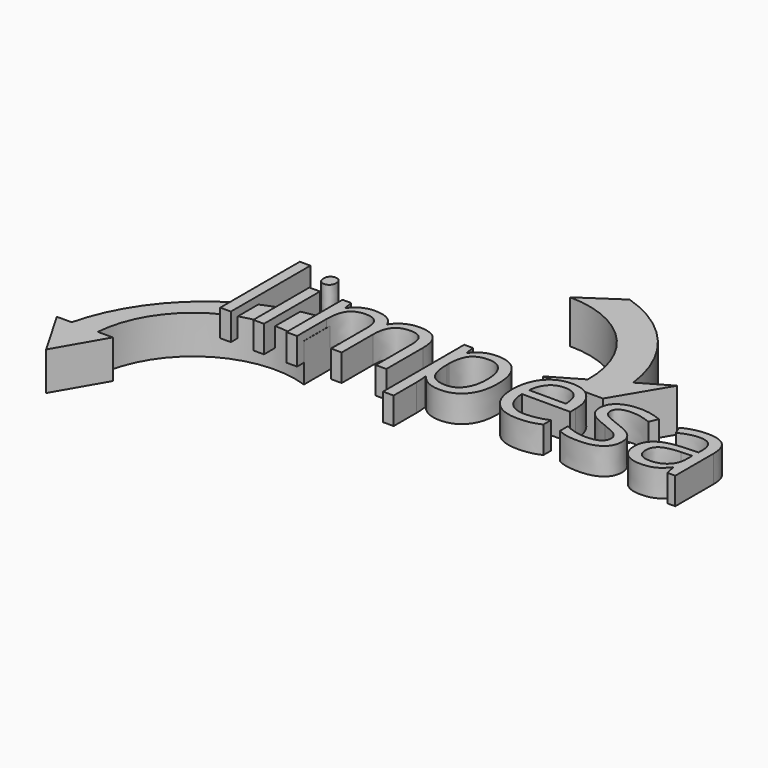
from build123d import *

# Parameters (mm, degrees)
F1_DEPTH     = 20
F3_DEPTH     = 17.82131
F4_TEXT_SIZE = 121.5147268441
F5_DEPTH     = 25


# Not quite as in the source:
# - Text() gives the source's letters only with a copy of the font that has no kerning and outlines rounded to 1/6400 em; it was checked with that copy


with BuildPart() as f1:
    # F0 (on Top) → F1 (new body, symmetric)
    with BuildSketch(Plane.XY):
        Polygon((90.5845264921, 157.8935082592), (62.1264589041, 141.4145874905), (117.9384660276, 141.4145874905), (147.349569231, 190.7638582515), (119.4569268128, 174.6123524257), align=None)
        with BuildLine():
            ThreePointArc((0, 250.6090158166), (64.810727857, 223.3211126078), (90.5845264921, 157.8935082592))
            Line((90.5845264921, 157.8935082592), (119.4569268128, 174.6123524257))
            ThreePointArc((119.4569268128, 174.6123524257), (92.4779303391, 237.015002481), (35.9874442945, 274.8406812071))
            Line((35.9874442945, 274.8406812071), (0, 250.6090158166))
        make_face()
    extrude(amount=F1_DEPTH, both=True)


with BuildPart() as f3:
    # F2 (on Top) → F3 (new body, symmetric)
    with BuildSketch(Plane.XY):
        Polygon((-260.2492953526, -2.3584535439), (-274.0066860809, -2.3584535439), (-248.0259239674, -47.3584535439), (-222.0451618538, -2.3584535439), (-236.0406206824, -2.3584535439), align=None)
        with BuildLine():
            ThreePointArc((-110.4163005948, 117.9332137108), (-205.6484047893, 83.0921104855), (-260.2492953526, -2.3584535439))
            Line((-260.2492953526, -2.3584535439), (-236.0406206824, -2.3584535439))
            ThreePointArc((-236.0406206824, -2.3584535439), (-193.4053290966, 69.5798529109), (-110.4163005948, 79.8613495194))
            Line((-110.4163005948, 79.8613495194), (-110.4163005948, 117.9332137108))
        make_face()
    extrude(amount=F3_DEPTH, both=True)

    # F4 (on Top) → F5 (join)
    with BuildSketch(Plane.XY):
        with Locations((-192.2960728407, 72.0282793045)):
            Text('limpesa', F4_TEXT_SIZE, font='Open Sans', text_align=(TextAlign.LEFT, TextAlign.BOTTOM))
    extrude(amount=F5_DEPTH)


solid = Compound([f1.part, f3.part])
